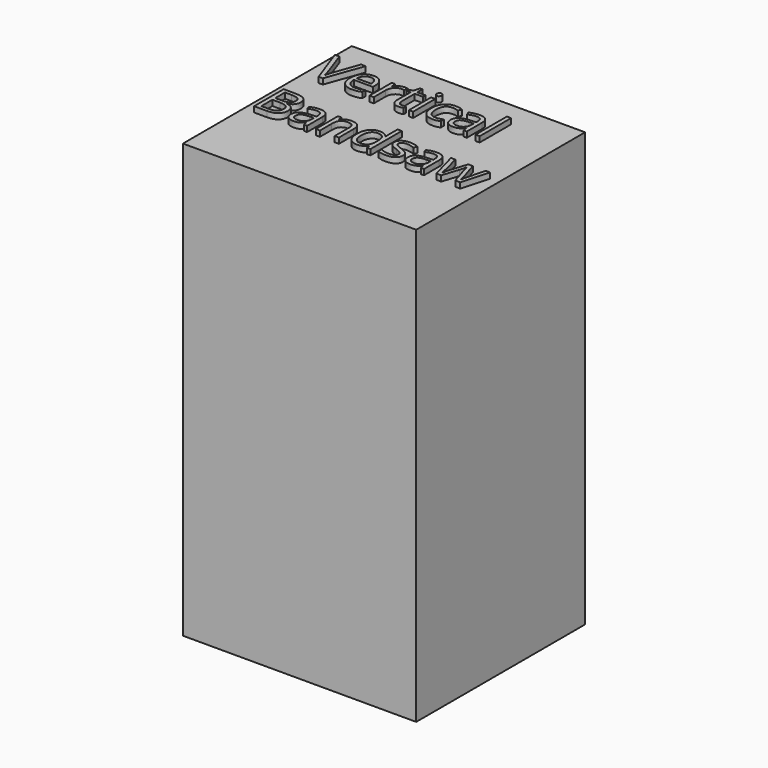
from build123d import *

# Parameters (mm, degrees)
F0_W         = 1066.8
F0_H         = 965.2
F1_DEPTH     = 1981.2
F2_TEXT_SIZE = 236.5197148261
F3_DEPTH     = 25.4


# Not quite as in the source:
# - Text() gives the source's letters only with a copy of the font that has no kerning and outlines rounded to 1/6400 em; it was checked with that copy


with BuildPart() as f1:
    # F0 (on Top) → F1 (new body)
    with BuildSketch(Plane.XY):
        Rectangle(F0_W, F0_H)
    extrude(amount=F1_DEPTH)

    # F2 (on face) → F3 (join)
    with BuildSketch(Plane.XY.offset(1981.2)):
        with Locations((-508, 185.3058053252)):
            Text('Vertical', F2_TEXT_SIZE, font='Open Sans', text_align=(TextAlign.LEFT, TextAlign.BOTTOM))
        with Locations((-508, -136.3610068384)):
            Text('Bandsaw', F2_TEXT_SIZE, font='Open Sans', text_align=(TextAlign.LEFT, TextAlign.BOTTOM))
    extrude(amount=F3_DEPTH)


solid = f1.part
